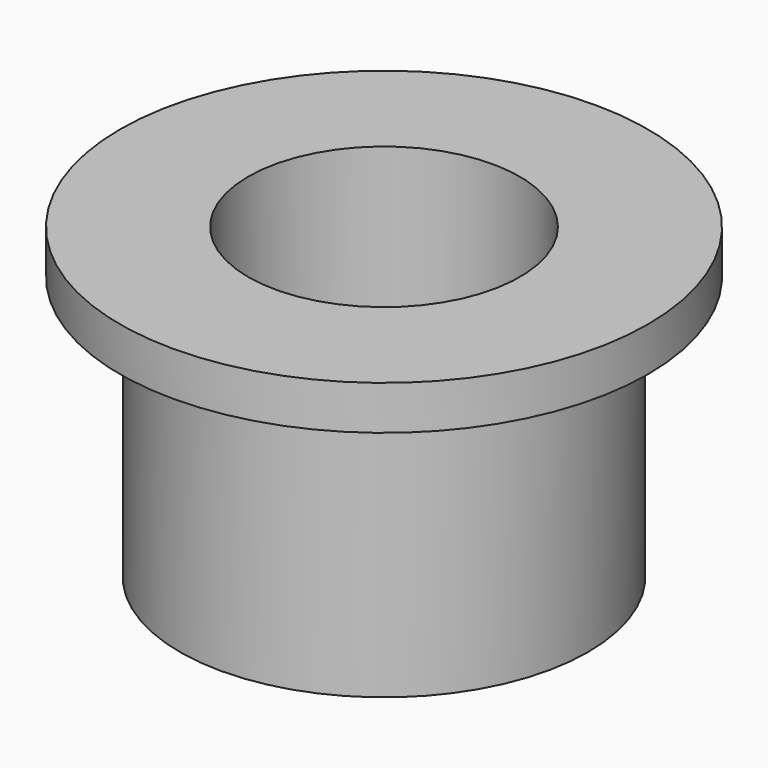
from build123d import *

# Parameters (mm, degrees)
F2_R     = 7.366
F3_DEPTH = 9.525
F4_R     = 9.525
F5_DEPTH = 1.5875
F8_D     = 9.8044


# Not quite as in the source:
# - a feature of the source that left no trace in its solid (it failed there, or was rolled back) is left out


with BuildPart() as f3:
    # F2 (on Top) → F3 (new body, through all)
    with BuildSketch(Plane.XY):
        Circle(F2_R)
    extrude(amount=-F3_DEPTH)

    # F4 (on Top) → F5 (join, through all)
    with BuildSketch(Plane.XY):
        Circle(F4_R)
    extrude(amount=F5_DEPTH)

    # F8 (through all)
    with Locations(Plane(origin=(0, 0, -9.525), x_dir=(1, 0, 0), z_dir=(0, 0, -1))):
        with Locations((0, 0)):
            Hole(F8_D / 2)


solid = f3.part
